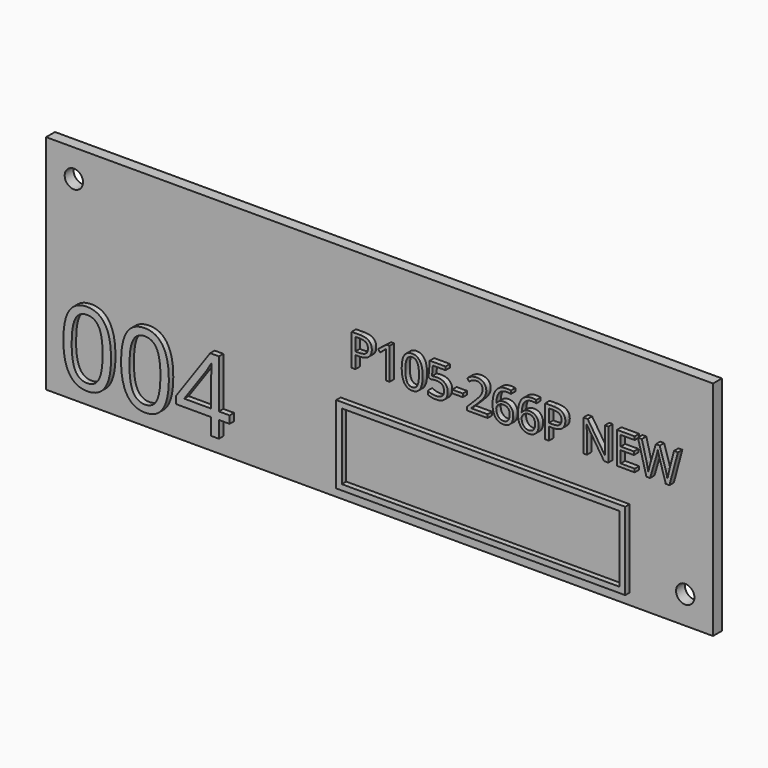
from build123d import *

# Parameters (mm, degrees)
F0_W         = 120
F0_H         = 40
F1_DEPTH     = 2
F3_D         = 3.3
F4_TEXT_SIZE = 7.9968345863
F5_DEPTH     = 1
F6_TEXT_SIZE = 18.1818181818
F7_DEPTH     = 1
F8_W         = 52
F8_H         = 14
F8_W_2       = 49.99999962
F8_H_2       = 11.99999962
F9_DEPTH     = 1


# Not quite as in the source:
# - Text() gives the source's letters only with a copy of the font that has no kerning and outlines rounded to 1/6400 em; it was checked with that copy


with BuildPart() as f1:
    # F0 (on Front) → F1 (new body)
    with BuildSketch(Plane.XZ):
        Rectangle(F0_W, F0_H)
    extrude(amount=F1_DEPTH)

    # F3 (through all)
    with Locations(Plane.XZ.offset(2)):
        with Locations((-55, 15), (55, -15)):
            Hole(F3_D / 2)

    # F4 (on face) → F5 (join)
    with BuildSketch(Plane.XZ.offset(2)):
        with Locations((-5, 2)):
            Text('P105-266P NEW', F4_TEXT_SIZE, font='Open Sans', text_align=(TextAlign.LEFT, TextAlign.BOTTOM))
    extrude(amount=F5_DEPTH)

    # F6 (on face) → F7 (join)
    with BuildSketch(Plane.XZ.offset(2)):
        with Locations((-57, -17)):
            Text('004', F6_TEXT_SIZE, font='Open Sans', text_align=(TextAlign.LEFT, TextAlign.BOTTOM))
    extrude(amount=F7_DEPTH)

    # F8 (on face) → F9 (join)
    with BuildSketch(Plane.XZ.offset(2)):
        with Locations((19, -11)):
            Rectangle(F8_W, F8_H)
        with Locations((19, -11)):
            Rectangle(F8_W_2, F8_H_2, mode=Mode.SUBTRACT)
    extrude(amount=F9_DEPTH)


solid = f1.part
